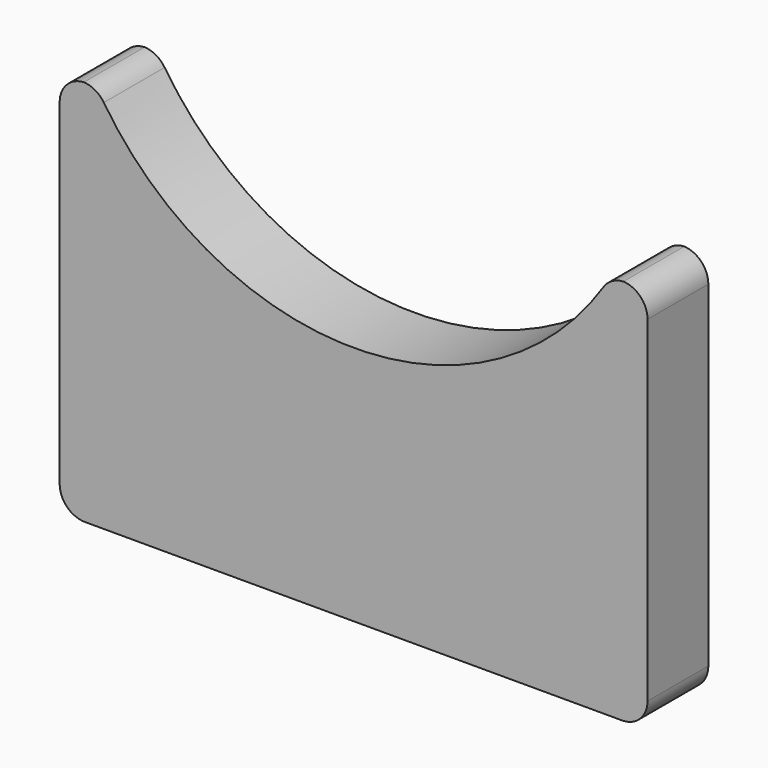
from build123d import *

# Parameters (mm, degrees)
F1_DEPTH    = 19.05
F2_T1_DEPTH = 50.8
F2_T3_DEPTH = 36.6217233344


# Not quite as in the source:
# - a fillet or chamfer that OpenCascade refuses, or shapes differently, is made with other operations: its cross-section is extruded or revolved along the edge and cut away or added


with BuildPart() as f1:
    # F0 (on Front) → F1 (new body)
    with BuildSketch(Plane.XZ):
        with BuildLine():
            ThreePointArc((64.3887874714, -38.322173059), (0, -74.93), (-64.3887874714, -38.322173059))
            Line((-64.3887874714, -38.322173059), (-73.66, -38.322173059))
            Line((-73.66, -38.322173059), (-73.66, -135.255))
            Line((-73.66, -135.255), (73.66, -135.255))
            Line((73.66, -135.255), (73.66, -38.322173059))
            Line((73.66, -38.322173059), (64.3887874714, -38.322173059))
        make_face()
    extrude(amount=F1_DEPTH)

    # F2: fillet of radius 6.35 on 6 edges, made by hand

    # F2_s2 → F2_t1 (cut)
    with BuildSketch(Plane.XZ.offset(-15.875)):
        with BuildLine():
            ThreePointArc((67.31, -38.322173059), (71.8001280605, -40.1820449985), (73.66, -44.672173059))
            Line((73.66, -44.672173059), (73.66, -38.322173059))
            Line((73.66, -38.322173059), (67.31, -38.322173059))
        make_face()
        with BuildLine():
            ThreePointArc((-67.31, -38.322173059), (-71.8001280605, -40.1820449985), (-73.66, -44.672173059))
            Line((-73.66, -44.672173059), (-73.66, -38.322173059))
            Line((-73.66, -38.322173059), (-67.31, -38.322173059))
        make_face()
        with BuildLine():
            ThreePointArc((67.31, -135.255), (71.8001280605, -133.3951280605), (73.66, -128.905))
            Line((73.66, -128.905), (73.66, -135.255))
            Line((73.66, -135.255), (67.31, -135.255))
        make_face()
        with BuildLine():
            ThreePointArc((-73.66, -128.905), (-71.8001280605, -133.3951280605), (-67.31, -135.255))
            Line((-67.31, -135.255), (-73.66, -135.255))
            Line((-73.66, -135.255), (-73.66, -128.905))
        make_face()
    extrude(amount=F2_T1_DEPTH, mode=Mode.SUBTRACT)

    # F2_s4 → F2_t3 (cut)
    with BuildSketch(Plane.XZ.offset(-8.7858616672)):
        with BuildLine():
            ThreePointArc((-62.59819994, -41.1821595388), (-64.889752462, -39.0827148628), (-67.9031321383, -38.322173059))
            Line((-67.9031321383, -38.322173059), (-64.3887874714, -38.322173059))
            ThreePointArc((-64.3887874714, -38.322173059), (-63.5095947367, -39.7622468729), (-62.59819994, -41.1821595388))
        make_face()
        with BuildLine():
            ThreePointArc((67.9031321383, -38.322173059), (64.889752462, -39.0827148628), (62.59819994, -41.1821595388))
            ThreePointArc((62.59819994, -41.1821595388), (63.5095947367, -39.7622468729), (64.3887874714, -38.322173059))
            Line((64.3887874714, -38.322173059), (67.9031321383, -38.322173059))
        make_face()
    extrude(amount=F2_T3_DEPTH, mode=Mode.SUBTRACT)


solid = f1.part
